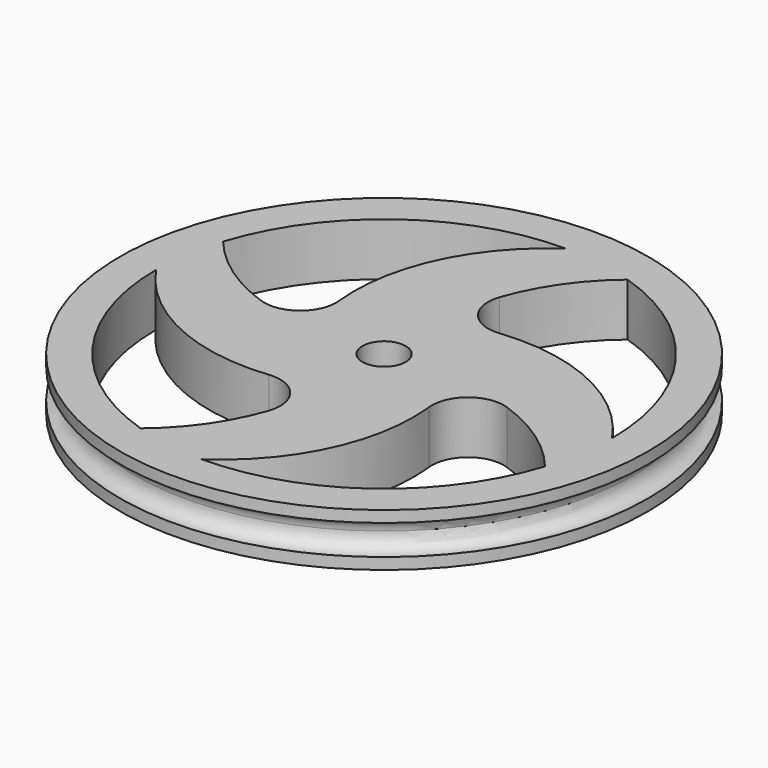
from build123d import *

# Parameters (mm, degrees)
F0_R     = 27.94
F0_R_2   = 2.286
F1_DEPTH = 2.794
F4_R     = 3.81
F5_DEPTH = 12.7


# Not quite as in the source:
# - a feature names something its author has since deleted; it is built from what else it names


with BuildPart() as f1:
    # F0 (on Top) → F1 (new body, symmetric)
    with BuildSketch(Plane.XY):
        Circle(F0_R)
        with BuildLine():
            ThreePointArc((7.4038372238, 22.9660639719), (19.5052748277, 14.2056732996), (24.13, 0))
            ThreePointArc((24.13, 0), (23.8372400211, -3.7473841781), (22.9660639719, -7.4038372238))
            ThreePointArc((22.9660639719, -7.4038372238), (14.2056732996, -19.5052748277), (0, -24.13))
            ThreePointArc((0, -24.13), (-3.7473841781, -23.8372400211), (-7.4038372238, -22.9660639719))
            ThreePointArc((-7.4038372238, -22.9660639719), (-19.5052748277, -14.2056732996), (-24.13, 0))
            ThreePointArc((-24.13, 0), (-23.8372400211, 3.7473841781), (-22.9660639719, 7.4038372238))
            ThreePointArc((-22.9660639719, 7.4038372238), (-14.2056732996, 19.5052748277), (0, 24.13))
            ThreePointArc((0, 24.13), (3.7473841781, 23.8372400211), (7.4038372238, 22.9660639719))
        make_face(mode=Mode.SUBTRACT)
        with BuildLine():
            ThreePointArc((22.9660639719, -7.4038372238), (23.8372400211, -3.7473841781), (24.13, 0))
            ThreePointArc((24.13, 0), (13.395886303, 8.0244732927), (0, 7.62))
            ThreePointArc((0, 7.62), (2.0157431704, 16.1065414645), (7.4038372238, 22.9660639719))
            ThreePointArc((7.4038372238, 22.9660639719), (3.7473841781, 23.8372400211), (0, 24.13))
            ThreePointArc((0, 24.13), (-8.0244732927, 13.395886303), (-7.62, 0))
            ThreePointArc((-7.62, 0), (-16.1065414645, 2.0157431704), (-22.9660639719, 7.4038372238))
            ThreePointArc((-22.9660639719, 7.4038372238), (-23.8372400211, 3.7473841781), (-24.13, 0))
            ThreePointArc((-24.13, 0), (-13.395886303, -8.0244732927), (0, -7.62))
            ThreePointArc((0, -7.62), (-2.0157431704, -16.1065414645), (-7.4038372238, -22.9660639719))
            ThreePointArc((-7.4038372238, -22.9660639719), (-3.7473841781, -23.8372400211), (0, -24.13))
            ThreePointArc((0, -24.13), (8.0244732927, -13.395886303), (7.62, 0))
            ThreePointArc((7.62, 0), (16.1065414645, -2.0157431704), (22.9660639719, -7.4038372238))
        make_face()
        Polygon((3.1270369256, 6.3063403068), (7.0249693735, 0.4450767373), (3.8979324478, -5.8612635696), (-3.1270369256, -6.3063403068), (-7.0249693735, -0.4450767373), (-3.8979324478, 5.8612635696), align=None, mode=Mode.SUBTRACT)
        Polygon((3.8979324478, -5.8612635696), (7.0249693735, 0.4450767373), (3.1270369256, 6.3063403068), (-3.8979324478, 5.8612635696), (-7.0249693735, -0.4450767373), (-3.1270369256, -6.3063403068), align=None)
        Circle(F0_R_2, mode=Mode.SUBTRACT)
    extrude(amount=F1_DEPTH, both=True)

    # F2 (on Front) → F3 (revolve, cut)
    with BuildSketch(Plane.XZ):
        with BuildLine():
            Line((27.94, -1.5875), (27.94, 0))
            Line((27.94, 0), (26.3525, 0))
            ThreePointArc((26.3525, 0), (26.8174679849, -1.1225320151), (27.94, -1.5875))
        make_face()
        with BuildLine():
            Line((26.3525, 0), (27.94, 0))
            Line((27.94, 0), (27.94, 1.5875))
            ThreePointArc((27.94, 1.5875), (26.8174679849, 1.1225320151), (26.3525, 0))
        make_face()
    revolve(axis=Axis((0, 0, -0.2561928704), (0, 0, -1)), mode=Mode.SUBTRACT)

    # F4
    f4_edges = [f1.edges().sort_by_distance(p)[0] for p in [
        (-7.62, 0, 0),
        (0, 7.62, 0),
        (7.62, 0, 0),
        (0, -7.62, 0),
    ]]
    fillet(f4_edges, radius=F4_R)

    # F0 (on Top) → F5 (cut)
    with BuildSketch(Plane.XY):
        Polygon((3.8979324478, -5.8612635696), (7.0249693735, 0.4450767373), (3.1270369256, 6.3063403068), (-3.8979324478, 5.8612635696), (-7.0249693735, -0.4450767373), (-3.1270369256, -6.3063403068), align=None)
        Circle(F0_R_2, mode=Mode.SUBTRACT)
    extrude(amount=-F5_DEPTH, mode=Mode.SUBTRACT)


solid = f1.part
